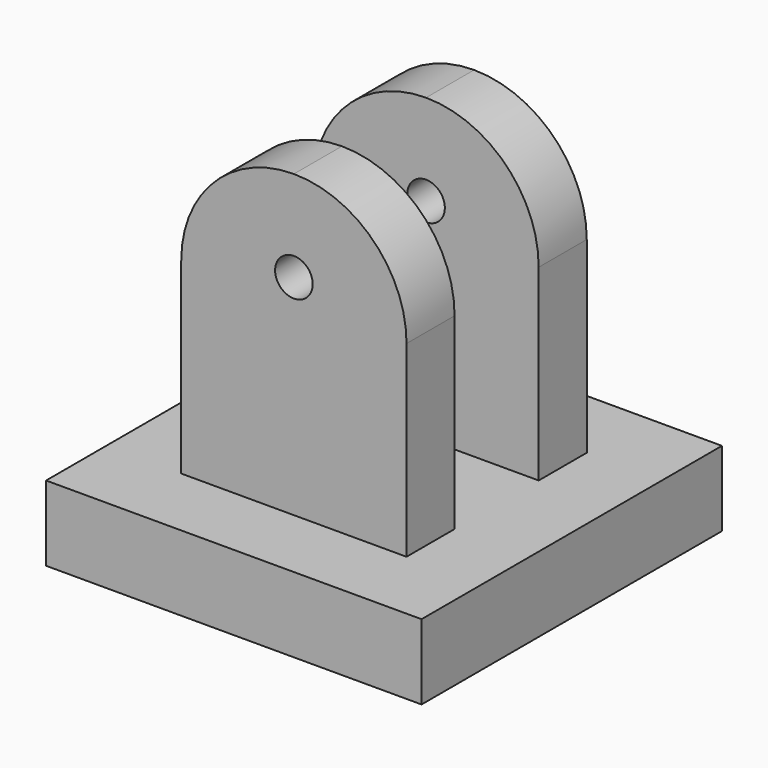
from build123d import *

# Parameters (mm, degrees)
F0_W     = 50
F0_H     = 50
F1_DEPTH = 10
F2_W     = 30
F2_H     = 8
F3_DEPTH = 40
F4_W     = 30
F4_H     = 8
F5_DEPTH = 40
F6_R     = 14.99999
F7_R     = 14.99999
F9_D     = 5


# Not quite as in the source:
# - a fillet or chamfer is up to 0.001 mm smaller than in the source, because OpenCascade refuses the exact size


with BuildPart() as f1:
    # F0 (on Top) → F1 (new body)
    with BuildSketch(Plane.XY):
        with Locations((1.1680303141, 2.4703653681)):
            Rectangle(F0_W, F0_H)
    extrude(amount=F1_DEPTH)

    # F2 (on face) → F3 (join)
    with BuildSketch(Plane.XY.offset(10)):
        with Locations((1.1680303141, -8.5296346319)):
            Rectangle(F2_W, F2_H)
    extrude(amount=F3_DEPTH)

    # F4 (on face) → F5 (join)
    with BuildSketch(Plane.XY.offset(10)):
        with Locations((1.1680303141, 13.4703653681)):
            Rectangle(F4_W, F4_H)
    extrude(amount=F5_DEPTH)

    # F6 (radius 15 in the source; OpenCascade refuses exactly that, so slightly less here)
    f6_edges = [f1.edges().sort_by_distance(p)[0] for p in [
        (-13.83197, -8.529635, 50),
        (16.16803, -8.529635, 50),
    ]]
    fillet(f6_edges, radius=F6_R)

    # F7 (radius 15 in the source; OpenCascade refuses exactly that, so slightly less here)
    f7_edges = [f1.edges().sort_by_distance(p)[0] for p in [
        (16.16803, 13.470365, 50),
        (-13.83197, 13.470365, 50),
    ]]
    fillet(f7_edges, radius=F7_R)

    # F9 (through all)
    with Locations(Plane.XZ.offset(12.5296346319)):
        with Locations((1.1680303141, 37.8934629261)):
            Hole(F9_D / 2)


solid = f1.part
